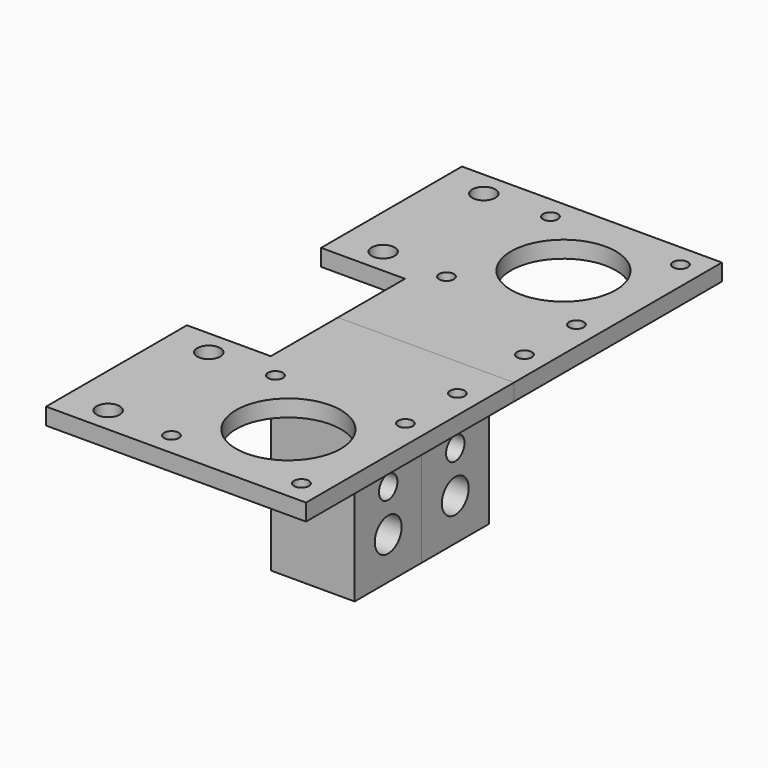
from build123d import *

# Parameters (mm, degrees)
F0_W      = 42
F0_H      = 42
F1_DEPTH  = 2
F2_R      = 1.75
F3_DEPTH  = 4.001
F4_DEPTH  = 20
F5_R      = 2.75
F6_DEPTH  = 4.001
F7_W      = 20
F7_H      = 45
F8_DEPTH  = 20
F9_DEPTH  = 20
F10_R     = 4
F10_R_2   = 2.75
F11_DEPTH = 40.001
F12_R     = 1.75
F13_DEPTH = 4.001
F14_R     = 12.5
F15_DEPTH = 4.001


with BuildPart() as f1:
    # F0 (on Top) → F1 (new body, symmetric)
    with BuildSketch(Plane.XY):
        Rectangle(F0_W, F0_H)
    extrude(amount=F1_DEPTH, both=True)

    # F2 (on face) → F3 (cut, through all)
    with BuildSketch(Plane.XY.offset(2)):
        with Locations((-15.5, 15.5)):
            Circle(F2_R)
        with Locations((15.5, 15.5)):
            Circle(F2_R)
        with Locations((-15.5, -15.5)):
            Circle(F2_R)
        with Locations((15.5, -15.5)):
            Circle(F2_R)
    extrude(amount=-F3_DEPTH, mode=Mode.SUBTRACT)

    # F4 (add): a face of the model
    f4_faces = [f1.faces().sort_by_distance(p)[0] for p in [
        (-21, 0, 0),
    ]]
    extrude(f4_faces, amount=F4_DEPTH)

    # F5 (on face) → F6 (cut, through all)
    with BuildSketch(Plane.XY.offset(2)):
        with Locations((-31, 15)):
            Circle(F5_R)
        with Locations((-31, -15)):
            Circle(F5_R)
    extrude(amount=-F6_DEPTH, mode=Mode.SUBTRACT)

    # F7 (on face) → F8 (join)
    with BuildSketch(Plane(origin=(0, 21, 0), x_dir=(-1, 0, 0), z_dir=(0, 1, 0))):
        with Locations((11, -20.5)):
            Rectangle(F7_W, F7_H)
    extrude(amount=F8_DEPTH)

    # F9 (add, through all): a face of the model
    f9_faces = [f1.faces().sort_by_distance(p)[0] for p in [
        (10, 21, 0),
    ]]
    extrude(f9_faces, amount=F9_DEPTH)

    # F10 (on face) → F11 (cut, through all)
    with BuildSketch(Plane.YZ.offset(-1)):
        with Locations((31, -33)):
            Circle(F10_R)
        with Locations((31, -23)):
            Circle(F10_R_2)
    extrude(amount=-F11_DEPTH, mode=Mode.SUBTRACT)

    # F12 (on face) → F13 (cut, through all)
    with BuildSketch(Plane(origin=(0, 0, -2), x_dir=(1, 0, 0), z_dir=(0, 0, -1))):
        with Locations((15.5, -31.0000000004)):
            Circle(F12_R)
    extrude(amount=-F13_DEPTH, mode=Mode.SUBTRACT)

    # F14 (on face) → F15 (cut, through all)
    with BuildSketch(Plane(origin=(0, 0, -2), x_dir=(1, 0, 0), z_dir=(0, 0, -1))):
        Circle(F14_R)
    extrude(amount=-F15_DEPTH, mode=Mode.SUBTRACT)


with BuildPart() as f16_1:
    # F16: instance of F1
    add(f1.part.mirror(Plane(origin=(-9.1295546559, 41, -18.6740890688), x_dir=(-1, 0, 0), z_dir=(0, 1, 0))))


solid = Compound([f1.part, f16_1.part])
